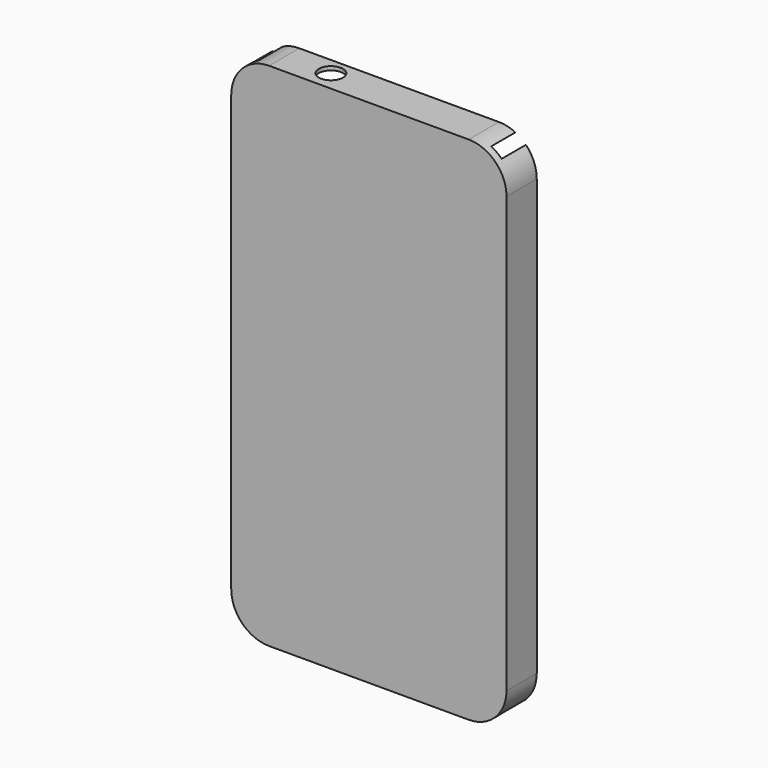
from build123d import *

# Parameters (mm, degrees)
F0_W      = 72.7374479175
F0_H      = 135
F1_DEPTH  = 10
F2_R      = 10
F3_W      = 67
F3_H      = 133
F4_DEPTH  = 8
F5_W      = 12.0182400569
F5_H      = 3.036568407
F6_DEPTH  = 25
F7_R      = 3.1730919104
F8_DEPTH  = 12
F9_W      = 2.8348967899
F9_H      = 53.2759986818
F10_DEPTH = 12


# Not quite as in the source:
# - a feature of the source that left no trace in its solid (it failed there, or was rolled back) is left out


with BuildPart() as f1:
    # F0 (on Front) → F1 (new body)
    with BuildSketch(Plane.XZ):
        Rectangle(F0_W, F0_H)
    extrude(amount=F1_DEPTH)

    # F2
    f2_edges = [f1.edges().sort_by_distance(p)[0] for p in [
        (36.368724, -5, 67.5),
        (-36.368724, -5, 67.5),
        (-36.368724, -5, -67.5),
        (36.368724, -5, -67.5),
    ]]
    fillet(f2_edges, radius=F2_R)

    # F3 (on Front) → F4 (cut)
    with BuildSketch(Plane.XZ):
        Rectangle(F3_W, F3_H)
    extrude(amount=F4_DEPTH, mode=Mode.SUBTRACT)

    # F5 (on face) → F6 (cut)
    with BuildSketch(Plane(origin=(0, 0, -67.5), x_dir=(1, 0, 0), z_dir=(0, 0, -1))):
        with Locations((-18.9633578993, 5.0012452994)):
            Rectangle(F5_W, F5_H)
    extrude(amount=-F6_DEPTH, mode=Mode.SUBTRACT)

    # F7 (on face) → F8 (cut)
    with BuildSketch(Plane.XY.offset(67.5)):
        with Locations((-14.315456152, -4.6320809051)):
            Circle(F7_R)
    extrude(amount=-F8_DEPTH, mode=Mode.SUBTRACT)

    # F9 (on face) → F10 (cut)
    with BuildSketch(Plane(origin=(-36.3687239587, 0, 0), x_dir=(0, -1, 0), z_dir=(-1, 0, 0))):
        with Locations((4.099019221, 26.6379993409)):
            Rectangle(F9_W, F9_H)
    extrude(amount=-F10_DEPTH, mode=Mode.SUBTRACT)


solid = f1.part
